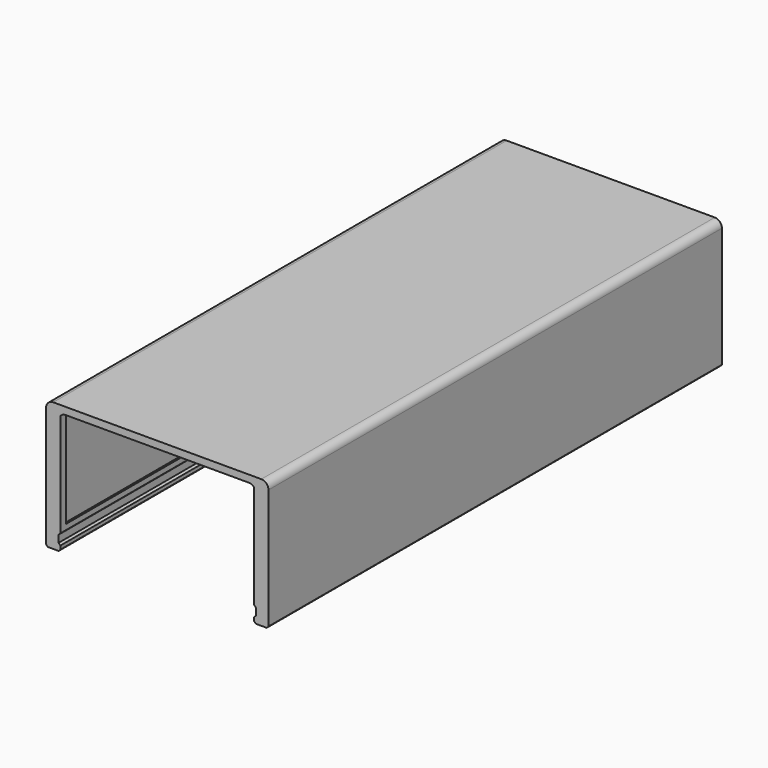
from build123d import *

# Parameters (mm, degrees)
F2_W     = 0.5
F2_H     = 2
F3_DEPTH = 79
F4_DEPTH = 77
F5_SIZE  = 0.49999


# Not quite as in the source:
# - a fillet or chamfer is up to 0.001 mm smaller than in the source, because OpenCascade refuses the exact size


with BuildPart() as f3:
    # F2 (on Front) → F3 (new body, symmetric)
    with BuildSketch(Plane.XZ):
        with BuildLine():
            Line((-27, -19), (-27, -17))
            Line((-27, -17), (-27.5, -17))
            Line((-27.5, -17), (-27.5, -15))
            Line((-27.5, -15), (-27.5, -13))
            Line((-27.5, -13), (-27.5, 13))
            Line((-27.5, 13), (-27.5, 15))
            Line((-27.5, 15), (-27, 15))
            Line((-27, 15), (-25.5, 15))
            Line((-25.5, 15), (0, 15))
            Line((0, 15), (25.5, 15))
            Line((25.5, 15), (27, 15))
            Line((27, 15), (27.5, 15))
            Line((27.5, 15), (27.5, 13))
            Line((27.5, 13), (27.5, -13))
            Line((27.5, -13), (27.5, -15))
            Line((27.5, -15), (27.5, -17))
            Line((27.5, -17), (27, -17))
            Line((27, -17), (27, -19))
            Line((27, -19), (31, -19))
            Line((31, -19), (31, 15))
            ThreePointArc((31, 15), (30.4142135624, 16.4142135624), (29, 17))
            Line((29, 17), (0, 17))
            Line((0, 17), (-29, 17))
            ThreePointArc((-29, 17), (-30.4142135624, 16.4142135624), (-31, 15))
            Line((-31, 15), (-31, -19))
            Line((-31, -19), (-27, -19))
        make_face()
        with Locations((-27.25, -14)):
            Rectangle(F2_W, F2_H)
        with BuildLine():
            Line((-27.5, 13), (-27.5, -13))
            Line((-27.5, -13), (-27, -13))
            Line((-27, -13), (-27, 14.3228756555))
            ThreePointArc((-27, 14.3228756555), (-27.3708286934, 13.7071067812), (-27.5, 13))
        make_face()
        with BuildLine():
            Line((-27.5, 15), (-27.5, 13))
            ThreePointArc((-27.5, 13), (-27.3708286934, 13.7071067812), (-27, 14.3228756555))
            Line((-27, 14.3228756555), (-27, 15))
            Line((-27, 15), (-27.5, 15))
        make_face()
        with BuildLine():
            Line((-27, 15), (-27, 14.3228756555))
            ThreePointArc((-27, 14.3228756555), (-26.3228756555, 14.8228756555), (-25.5, 15))
            Line((-25.5, 15), (-27, 15))
        make_face()
        with BuildLine():
            Line((27, 15), (25.5, 15))
            ThreePointArc((25.5, 15), (26.3228756555, 14.8228756555), (27, 14.3228756555))
            Line((27, 14.3228756555), (27, 15))
        make_face()
        with BuildLine():
            Line((27.5, 15), (27, 15))
            Line((27, 15), (27, 14.3228756555))
            ThreePointArc((27, 14.3228756555), (27.3708286934, 13.7071067812), (27.5, 13))
            Line((27.5, 13), (27.5, 15))
        make_face()
        with BuildLine():
            ThreePointArc((27.5, 13), (27.3708286934, 13.7071067812), (27, 14.3228756555))
            Line((27, 14.3228756555), (27, -13))
            Line((27, -13), (27.5, -13))
            Line((27.5, -13), (27.5, 13))
        make_face()
        with Locations((27.25, -14)):
            Rectangle(F2_W, F2_H)
    extrude(amount=F3_DEPTH, both=True)

    # F2 (on Front) → F4 (cut, symmetric)
    with BuildSketch(Plane.XZ):
        with BuildLine():
            Line((-27.5, 13), (-27.5, -13))
            Line((-27.5, -13), (-27, -13))
            Line((-27, -13), (-27, 14.3228756555))
            ThreePointArc((-27, 14.3228756555), (-27.3708286934, 13.7071067812), (-27.5, 13))
        make_face()
        with BuildLine():
            Line((-27.5, 15), (-27.5, 13))
            ThreePointArc((-27.5, 13), (-27.3708286934, 13.7071067812), (-27, 14.3228756555))
            Line((-27, 14.3228756555), (-27, 15))
            Line((-27, 15), (-27.5, 15))
        make_face()
        with BuildLine():
            ThreePointArc((27.5, 13), (27.3708286934, 13.7071067812), (27, 14.3228756555))
            Line((27, 14.3228756555), (27, -13))
            Line((27, -13), (27.5, -13))
            Line((27.5, -13), (27.5, 13))
        make_face()
    extrude(amount=F4_DEPTH, both=True, mode=Mode.SUBTRACT)

    # F5 (size 0.5 in the source; OpenCascade refuses exactly that, so slightly less here)
    f5_edges = [f3.edges().sort_by_distance(p)[0] for p in [
        (-27, 0, -17),
        (-27, 0, -15),
        (27, 0, -15),
        (27, 0, -17),
        (-27, 0, -19),
        (27, 0, -19),
        (-31, 0, -19),
        (31, 0, -19),
    ]]
    chamfer(f5_edges, length=F5_SIZE)


solid = f3.part
